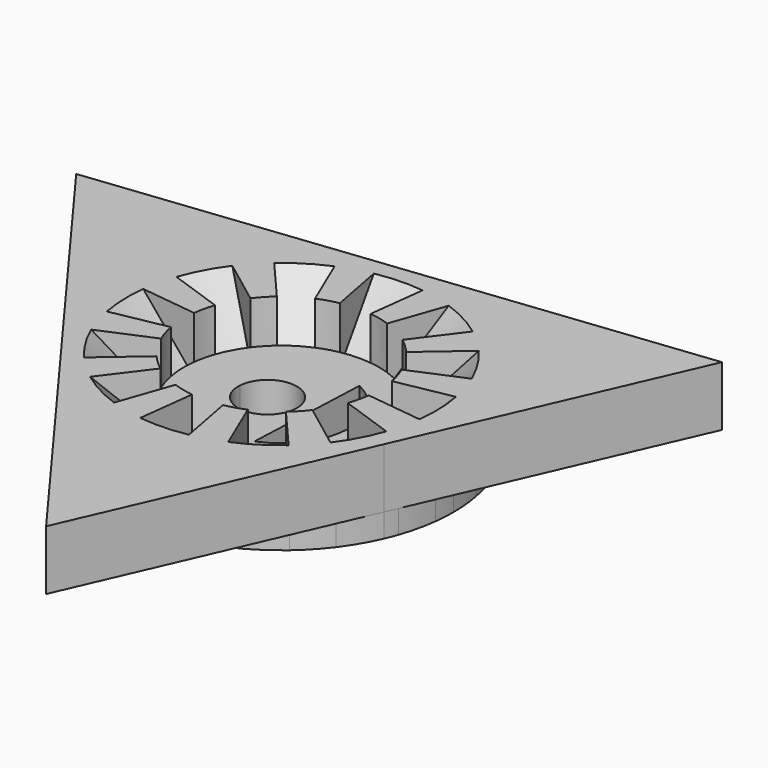
from build123d import *

# Parameters (mm, degrees)
F0_R     = 8.3058
F1_DEPTH = 5.08
F2_SIZE  = 4.826
F4_DEPTH = 5.08
F5_DEPTH = 1.4
F6_DEPTH = 2
F8_DEPTH = 25.4


# Not quite as in the source:
# - a feature names something its author has since deleted; it is built from what else it names


with BuildPart() as f1:
    # F0 (on Top) → F1 (new body)
    with BuildSketch(Plane.XY):
        with BuildLine():
            ThreePointArc((-11.7963555107, -8.6970380191), (-13.4300332581, 5.8674253575), (-1.6336763226, 14.564462754))
            Line((-1.6336763226, 14.564462754), (-26.8600673835, 11.7348487299))
            Line((-26.8600673835, 11.7348487299), (-11.7963555107, -8.6970380191))
        make_face()
        with BuildLine():
            Line((3.2673565821, -29.1289250664), (13.4300329735, -5.8674260091))
            ThreePointArc((13.4300329735, -5.8674260091), (1.6336773074, -14.5644626435), (-11.7963555107, -8.6970380191))
            Line((-11.7963555107, -8.6970380191), (3.2673565821, -29.1289250664))
        make_face()
        with BuildLine():
            ThreePointArc((13.4300329735, -5.8674260091), (14.3460857186, -2.9970482468), (14.6558, 0))
            ThreePointArc((14.6558, 0), (9.768562847, 10.9255504916), (-1.6336763226, 14.564462754))
            ThreePointArc((-1.6336763226, 14.564462754), (-13.4300332581, 5.8674253575), (-11.7963555107, -8.6970380191))
            ThreePointArc((-11.7963555107, -8.6970380191), (1.6336773074, -14.5644626435), (13.4300329735, -5.8674260091))
        make_face()
        Circle(F0_R, mode=Mode.SUBTRACT)
        with BuildLine():
            ThreePointArc((-1.6336763226, 14.564462754), (9.768562847, 10.9255504916), (14.6558, 0))
            ThreePointArc((14.6558, 0), (14.3460857186, -2.9970482468), (13.4300329735, -5.8674260091))
            Line((13.4300329735, -5.8674260091), (23.5927108014, 17.3940763365))
            Line((23.5927108014, 17.3940763365), (-1.6336763226, 14.564462754))
        make_face()
    extrude(amount=F1_DEPTH)

    # F2
    f2_edges = [f1.edges().sort_by_distance(p)[0] for p in [
        (-8.3058, 0, 5.08),
    ]]
    chamfer(f2_edges, length=F2_SIZE)

    # F3 (on face) → F4 (join, through all)
    with BuildSketch(Plane(origin=(0, 0, 0), x_dir=(1, 0, 0), z_dir=(0, 0, -1))):
        with BuildLine():
            ThreePointArc((-8.8120829317, 11.710664714), (-10.0148960998, 10.7002023229), (-11.1026461201, 9.5668031636))
            Line((-11.1026461201, 9.5668031636), (-6.2921408688, 5.4217411343))
            ThreePointArc((-6.2921408688, 5.4217411343), (-5.6756863512, 6.0640661345), (-4.994022736, 6.6367198639))
            Line((-4.994022736, 6.6367198639), (-8.8120829317, 11.710664714))
        make_face()
        with BuildLine():
            ThreePointArc((-2.7382832694, 7.8414359894), (-1.8832554968, 8.0894784983), (-1.0065906245, 8.244579368))
            Line((-1.0065906245, 8.244579368), (-1.7761553221, 14.5477746034))
            ThreePointArc((-1.7761553221, 14.5477746034), (-3.3230532772, 14.2740950871), (-4.8317720074, 13.8364176328))
            Line((-4.8317720074, 13.8364176328), (-2.7382832694, 7.8414359894))
        make_face()
        with BuildLine():
            ThreePointArc((1.5492951207, 8.1600244037), (2.4137921471, 7.9473216313), (3.250556632, 7.6433104884))
            Line((3.250556632, 7.6433104884), (5.7356916717, 13.4868200361))
            ThreePointArc((5.7356916717, 13.4868200361), (4.2591989874, 14.0232556001), (2.7337715126, 14.3985751711))
            Line((2.7337715126, 14.3985751711), (1.5492951207, 8.1600244037))
        make_face()
        with BuildLine():
            ThreePointArc((5.4217411343, 6.2921408688), (6.0640661345, 5.6756863512), (6.6367198639, 4.994022736))
            Line((6.6367198639, 4.994022736), (11.710664714, 8.8120829317))
            ThreePointArc((11.710664714, 8.8120829317), (10.7002023229, 10.0148960998), (9.5668031636, 11.1026461201))
            Line((9.5668031636, 11.1026461201), (5.4217411343, 6.2921408688))
        make_face()
        with BuildLine():
            ThreePointArc((7.8414359894, 2.7382832694), (8.0894784983, 1.8832554968), (8.244579368, 1.0065906245))
            Line((8.244579368, 1.0065906245), (14.5477746034, 1.7761553221))
            ThreePointArc((14.5477746034, 1.7761553221), (14.2740950871, 3.3230532772), (13.8364176328, 4.8317720074))
            Line((13.8364176328, 4.8317720074), (7.8414359894, 2.7382832694))
        make_face()
        with BuildLine():
            Line((14.3985751711, -2.7337715126), (8.1600244037, -1.5492951207))
            ThreePointArc((8.1600244037, -1.5492951207), (7.9473216313, -2.4137921471), (7.6433104884, -3.250556632))
            Line((7.6433104884, -3.250556632), (13.4868200361, -5.7356916717))
            ThreePointArc((13.4868200361, -5.7356916717), (14.0232556001, -4.2591989874), (14.3985751711, -2.7337715126))
        make_face()
        with BuildLine():
            Line((11.1026461201, -9.5668031636), (6.2921408688, -5.4217411343))
            ThreePointArc((6.2921408688, -5.4217411343), (5.6756863512, -6.0640661345), (4.994022736, -6.6367198639))
            Line((4.994022736, -6.6367198639), (8.8120829317, -11.710664714))
            ThreePointArc((8.8120829317, -11.710664714), (10.0148960998, -10.7002023229), (11.1026461201, -9.5668031636))
        make_face()
        with BuildLine():
            Line((4.8317720074, -13.8364176328), (2.7382832694, -7.8414359894))
            ThreePointArc((2.7382832694, -7.8414359894), (1.8832554968, -8.0894784983), (1.0065906245, -8.244579368))
            Line((1.0065906245, -8.244579368), (1.7761553221, -14.5477746034))
            ThreePointArc((1.7761553221, -14.5477746034), (3.3230532772, -14.2740950871), (4.8317720074, -13.8364176328))
        make_face()
        with BuildLine():
            ThreePointArc((-1.5492951207, -8.1600244037), (-2.4137921471, -7.9473216313), (-3.250556632, -7.6433104884))
            Line((-3.250556632, -7.6433104884), (-5.7356916717, -13.4868200361))
            ThreePointArc((-5.7356916717, -13.4868200361), (-4.2591989874, -14.0232556001), (-2.7337715126, -14.3985751711))
            Line((-2.7337715126, -14.3985751711), (-1.5492951207, -8.1600244037))
        make_face()
        with BuildLine():
            Line((-9.5668031636, -11.1026461201), (-5.4217411343, -6.2921408688))
            ThreePointArc((-5.4217411343, -6.2921408688), (-6.0640661345, -5.6756863512), (-6.6367198639, -4.994022736))
            Line((-6.6367198639, -4.994022736), (-11.710664714, -8.8120829317))
            ThreePointArc((-11.710664714, -8.8120829317), (-10.7002023229, -10.0148960998), (-9.5668031636, -11.1026461201))
        make_face()
        with BuildLine():
            Line((-13.8364176328, -4.8317720074), (-7.8414359894, -2.7382832694))
            ThreePointArc((-7.8414359894, -2.7382832694), (-8.0894784983, -1.8832554968), (-8.244579368, -1.0065906245))
            Line((-8.244579368, -1.0065906245), (-14.5477746034, -1.7761553221))
            ThreePointArc((-14.5477746034, -1.7761553221), (-14.2740950871, -3.3230532772), (-13.8364176328, -4.8317720074))
        make_face()
        with BuildLine():
            Line((-7.6433104884, 3.250556632), (-13.4868200361, 5.7356916717))
            ThreePointArc((-13.4868200361, 5.7356916717), (-14.0232556001, 4.2591989874), (-14.3985751711, 2.7337715126))
            Line((-14.3985751711, 2.7337715126), (-8.1600244037, 1.5492951207))
            ThreePointArc((-8.1600244037, 1.5492951207), (-7.9473216313, 2.4137921471), (-7.6433104884, 3.250556632))
        make_face()
    extrude(amount=-F4_DEPTH)


with BuildPart() as f5:
    # F3 (on face) → F5 (new body)
    with BuildSketch(Plane(origin=(0, 0, 0), x_dir=(1, 0, 0), z_dir=(0, 0, -1))):
        with BuildLine():
            ThreePointArc((8.1600244037, -1.5492951207), (8.2692757945, -0.7780690675), (8.3058, 0))
            ThreePointArc((8.3058, 0), (8.2904807145, 0.5042253095), (8.244579368, 1.0065906245))
            ThreePointArc((8.244579368, 1.0065906245), (8.0894784983, 1.8832554968), (7.8414359894, 2.7382832694))
            ThreePointArc((7.8414359894, 2.7382832694), (7.3264138133, 3.9127962221), (6.6367198639, 4.994022736))
            ThreePointArc((6.6367198639, 4.994022736), (6.0640661345, 5.6756863512), (5.4217411343, 6.2921408688))
            ThreePointArc((5.4217411343, 6.2921408688), (4.3884623699, 7.0517878349), (3.250556632, 7.6433104884))
            Line((3.250556632, 7.6433104884), (-3.250556632, -7.6433104884))
            ThreePointArc((-3.250556632, -7.6433104884), (-2.4137921471, -7.9473216313), (-1.5492951207, -8.1600244037))
            ThreePointArc((-1.5492951207, -8.1600244037), (-0.2746259785, -8.301258592), (1.0065906245, -8.244579368))
            ThreePointArc((1.0065906245, -8.244579368), (1.8832554968, -8.0894784983), (2.7382832694, -7.8414359894))
            ThreePointArc((2.7382832694, -7.8414359894), (3.9127962221, -7.3264138133), (4.994022736, -6.6367198639))
            ThreePointArc((4.994022736, -6.6367198639), (5.6756863512, -6.0640661345), (6.2921408688, -5.4217411343))
            ThreePointArc((6.2921408688, -5.4217411343), (7.0517878349, -4.3884623699), (7.6433104884, -3.250556632))
            ThreePointArc((7.6433104884, -3.250556632), (7.9473216313, -2.4137921471), (8.1600244037, -1.5492951207))
        make_face()
        with BuildLine():
            Line((-3.250556632, -7.6433104884), (3.250556632, 7.6433104884))
            ThreePointArc((3.250556632, 7.6433104884), (2.4137921471, 7.9473216313), (1.5492951207, 8.1600244037))
            ThreePointArc((1.5492951207, 8.1600244037), (0.2746259785, 8.301258592), (-1.0065906245, 8.244579368))
            ThreePointArc((-1.0065906245, 8.244579368), (-1.8832554968, 8.0894784983), (-2.7382832694, 7.8414359894))
            ThreePointArc((-2.7382832694, 7.8414359894), (-3.9127962221, 7.3264138133), (-4.994022736, 6.6367198639))
            ThreePointArc((-4.994022736, 6.6367198639), (-5.6756863512, 6.0640661345), (-6.2921408688, 5.4217411343))
            ThreePointArc((-6.2921408688, 5.4217411343), (-7.0517878349, 4.3884623699), (-7.6433104884, 3.250556632))
            ThreePointArc((-7.6433104884, 3.250556632), (-7.9473216313, 2.4137921471), (-8.1600244037, 1.5492951207))
            ThreePointArc((-8.1600244037, 1.5492951207), (-8.301258592, 0.2746259785), (-8.244579368, -1.0065906245))
            ThreePointArc((-8.244579368, -1.0065906245), (-8.0894784983, -1.8832554968), (-7.8414359894, -2.7382832694))
            ThreePointArc((-7.8414359894, -2.7382832694), (-7.3264138133, -3.9127962221), (-6.6367198639, -4.994022736))
            ThreePointArc((-6.6367198639, -4.994022736), (-6.0640661345, -5.6756863512), (-5.4217411343, -6.2921408688))
            ThreePointArc((-5.4217411343, -6.2921408688), (-4.3884623699, -7.0517878349), (-3.250556632, -7.6433104884))
        make_face()
    extrude(amount=-F5_DEPTH)

    # F3 (on face) → F6 (join)
    with BuildSketch(Plane(origin=(0, 0, 0), x_dir=(1, 0, 0), z_dir=(0, 0, -1))):
        with BuildLine():
            ThreePointArc((8.1600244037, -1.5492951207), (8.2692757945, -0.7780690675), (8.3058, 0))
            ThreePointArc((8.3058, 0), (8.2904807145, 0.5042253095), (8.244579368, 1.0065906245))
            ThreePointArc((8.244579368, 1.0065906245), (8.0894784983, 1.8832554968), (7.8414359894, 2.7382832694))
            ThreePointArc((7.8414359894, 2.7382832694), (7.3264138133, 3.9127962221), (6.6367198639, 4.994022736))
            ThreePointArc((6.6367198639, 4.994022736), (6.0640661345, 5.6756863512), (5.4217411343, 6.2921408688))
            ThreePointArc((5.4217411343, 6.2921408688), (4.3884623699, 7.0517878349), (3.250556632, 7.6433104884))
            Line((3.250556632, 7.6433104884), (-3.250556632, -7.6433104884))
            ThreePointArc((-3.250556632, -7.6433104884), (-2.4137921471, -7.9473216313), (-1.5492951207, -8.1600244037))
            ThreePointArc((-1.5492951207, -8.1600244037), (-0.2746259785, -8.301258592), (1.0065906245, -8.244579368))
            ThreePointArc((1.0065906245, -8.244579368), (1.8832554968, -8.0894784983), (2.7382832694, -7.8414359894))
            ThreePointArc((2.7382832694, -7.8414359894), (3.9127962221, -7.3264138133), (4.994022736, -6.6367198639))
            ThreePointArc((4.994022736, -6.6367198639), (5.6756863512, -6.0640661345), (6.2921408688, -5.4217411343))
            ThreePointArc((6.2921408688, -5.4217411343), (7.0517878349, -4.3884623699), (7.6433104884, -3.250556632))
            ThreePointArc((7.6433104884, -3.250556632), (7.9473216313, -2.4137921471), (8.1600244037, -1.5492951207))
        make_face()
        with BuildLine():
            ThreePointArc((8.244579368, 1.0065906245), (8.2904807145, 0.5042253095), (8.3058, 0))
            ThreePointArc((8.3058, 0), (8.2692757945, -0.7780690675), (8.1600244037, -1.5492951207))
            Line((8.1600244037, -1.5492951207), (14.3985751711, -2.7337715126))
            ThreePointArc((14.3985751711, -2.7337715126), (14.5913520901, -1.3729230947), (14.6558, 0))
            ThreePointArc((14.6558, 0), (14.6287687225, 0.8897186654), (14.5477746034, 1.7761553221))
            Line((14.5477746034, 1.7761553221), (8.244579368, 1.0065906245))
        make_face()
        with BuildLine():
            ThreePointArc((7.8414359894, 2.7382832694), (8.0894784983, 1.8832554968), (8.244579368, 1.0065906245))
            Line((8.244579368, 1.0065906245), (14.5477746034, 1.7761553221))
            ThreePointArc((14.5477746034, 1.7761553221), (14.2740950871, 3.3230532772), (13.8364176328, 4.8317720074))
            Line((13.8364176328, 4.8317720074), (7.8414359894, 2.7382832694))
        make_face()
        with BuildLine():
            Line((14.3985751711, -2.7337715126), (8.1600244037, -1.5492951207))
            ThreePointArc((8.1600244037, -1.5492951207), (7.9473216313, -2.4137921471), (7.6433104884, -3.250556632))
            Line((7.6433104884, -3.250556632), (13.4868200361, -5.7356916717))
            ThreePointArc((13.4868200361, -5.7356916717), (14.0232556001, -4.2591989874), (14.3985751711, -2.7337715126))
        make_face()
        with BuildLine():
            ThreePointArc((6.6367198639, 4.994022736), (7.3264138133, 3.9127962221), (7.8414359894, 2.7382832694))
            Line((7.8414359894, 2.7382832694), (13.8364176328, 4.8317720074))
            ThreePointArc((13.8364176328, 4.8317720074), (13.6430563329, 5.3534556632), (13.4300337073, 5.8674243295))
            ThreePointArc((13.4300337073, 5.8674243295), (12.6562803718, 7.3899283347), (11.710664714, 8.8120829317))
            Line((11.710664714, 8.8120829317), (6.6367198639, 4.994022736))
        make_face()
        with BuildLine():
            Line((13.4868200361, -5.7356916717), (7.6433104884, -3.250556632))
            ThreePointArc((7.6433104884, -3.250556632), (7.0517878349, -4.3884623699), (6.2921408688, -5.4217411343))
            Line((6.2921408688, -5.4217411343), (11.1026461201, -9.5668031636))
            ThreePointArc((11.1026461201, -9.5668031636), (12.443062938, -7.7435559249), (13.4868200361, -5.7356916717))
        make_face()
        with BuildLine():
            ThreePointArc((5.4217411343, 6.2921408688), (6.0640661345, 5.6756863512), (6.6367198639, 4.994022736))
            Line((6.6367198639, 4.994022736), (11.710664714, 8.8120829317))
            ThreePointArc((11.710664714, 8.8120829317), (10.7002023229, 10.0148960998), (9.5668031636, 11.1026461201))
            Line((9.5668031636, 11.1026461201), (5.4217411343, 6.2921408688))
        make_face()
        with BuildLine():
            Line((11.1026461201, -9.5668031636), (6.2921408688, -5.4217411343))
            ThreePointArc((6.2921408688, -5.4217411343), (5.6756863512, -6.0640661345), (4.994022736, -6.6367198639))
            Line((4.994022736, -6.6367198639), (8.8120829317, -11.710664714))
            ThreePointArc((8.8120829317, -11.710664714), (10.0148960998, -10.7002023229), (11.1026461201, -9.5668031636))
        make_face()
        with BuildLine():
            ThreePointArc((3.250556632, 7.6433104884), (4.3884623699, 7.0517878349), (5.4217411343, 6.2921408688))
            Line((5.4217411343, 6.2921408688), (9.5668031636, 11.1026461201))
            ThreePointArc((9.5668031636, 11.1026461201), (7.7435559249, 12.443062938), (5.7356916717, 13.4868200361))
            Line((5.7356916717, 13.4868200361), (3.250556632, 7.6433104884))
        make_face()
        with BuildLine():
            Line((8.8120829317, -11.710664714), (4.994022736, -6.6367198639))
            ThreePointArc((4.994022736, -6.6367198639), (3.9127962221, -7.3264138133), (2.7382832694, -7.8414359894))
            Line((2.7382832694, -7.8414359894), (4.8317720074, -13.8364176328))
            ThreePointArc((4.8317720074, -13.8364176328), (6.9042306427, -12.9276476156), (8.8120829317, -11.710664714))
        make_face()
        with BuildLine():
            Line((-3.250556632, -7.6433104884), (3.250556632, 7.6433104884))
            ThreePointArc((3.250556632, 7.6433104884), (2.4137921471, 7.9473216313), (1.5492951207, 8.1600244037))
            ThreePointArc((1.5492951207, 8.1600244037), (0.2746259785, 8.301258592), (-1.0065906245, 8.244579368))
            ThreePointArc((-1.0065906245, 8.244579368), (-1.8832554968, 8.0894784983), (-2.7382832694, 7.8414359894))
            ThreePointArc((-2.7382832694, 7.8414359894), (-3.9127962221, 7.3264138133), (-4.994022736, 6.6367198639))
            ThreePointArc((-4.994022736, 6.6367198639), (-5.6756863512, 6.0640661345), (-6.2921408688, 5.4217411343))
            ThreePointArc((-6.2921408688, 5.4217411343), (-7.0517878349, 4.3884623699), (-7.6433104884, 3.250556632))
            ThreePointArc((-7.6433104884, 3.250556632), (-7.9473216313, 2.4137921471), (-8.1600244037, 1.5492951207))
            ThreePointArc((-8.1600244037, 1.5492951207), (-8.301258592, 0.2746259785), (-8.244579368, -1.0065906245))
            ThreePointArc((-8.244579368, -1.0065906245), (-8.0894784983, -1.8832554968), (-7.8414359894, -2.7382832694))
            ThreePointArc((-7.8414359894, -2.7382832694), (-7.3264138133, -3.9127962221), (-6.6367198639, -4.994022736))
            ThreePointArc((-6.6367198639, -4.994022736), (-6.0640661345, -5.6756863512), (-5.4217411343, -6.2921408688))
            ThreePointArc((-5.4217411343, -6.2921408688), (-4.3884623699, -7.0517878349), (-3.250556632, -7.6433104884))
        make_face()
        with BuildLine():
            ThreePointArc((1.5492951207, 8.1600244037), (2.4137921471, 7.9473216313), (3.250556632, 7.6433104884))
            Line((3.250556632, 7.6433104884), (5.7356916717, 13.4868200361))
            ThreePointArc((5.7356916717, 13.4868200361), (4.2591989874, 14.0232556001), (2.7337715126, 14.3985751711))
            Line((2.7337715126, 14.3985751711), (1.5492951207, 8.1600244037))
        make_face()
        with BuildLine():
            Line((4.8317720074, -13.8364176328), (2.7382832694, -7.8414359894))
            ThreePointArc((2.7382832694, -7.8414359894), (1.8832554968, -8.0894784983), (1.0065906245, -8.244579368))
            Line((1.0065906245, -8.244579368), (1.7761553221, -14.5477746034))
            ThreePointArc((1.7761553221, -14.5477746034), (3.3230532772, -14.2740950871), (4.8317720074, -13.8364176328))
        make_face()
        with BuildLine():
            ThreePointArc((-1.0065906245, 8.244579368), (0.2746259785, 8.301258592), (1.5492951207, 8.1600244037))
            Line((1.5492951207, 8.1600244037), (2.7337715126, 14.3985751711))
            ThreePointArc((2.7337715126, 14.3985751711), (0.4845846776, 14.6477865676), (-1.7761553221, 14.5477746034))
            Line((-1.7761553221, 14.5477746034), (-1.0065906245, 8.244579368))
        make_face()
        with BuildLine():
            Line((-5.7356916717, -13.4868200361), (-3.250556632, -7.6433104884))
            ThreePointArc((-3.250556632, -7.6433104884), (-4.3884623699, -7.0517878349), (-5.4217411343, -6.2921408688))
            Line((-5.4217411343, -6.2921408688), (-9.5668031636, -11.1026461201))
            ThreePointArc((-9.5668031636, -11.1026461201), (-7.7435559249, -12.443062938), (-5.7356916717, -13.4868200361))
        make_face()
        with BuildLine():
            ThreePointArc((-1.5492951207, -8.1600244037), (-2.4137921471, -7.9473216313), (-3.250556632, -7.6433104884))
            Line((-3.250556632, -7.6433104884), (-5.7356916717, -13.4868200361))
            ThreePointArc((-5.7356916717, -13.4868200361), (-4.2591989874, -14.0232556001), (-2.7337715126, -14.3985751711))
            Line((-2.7337715126, -14.3985751711), (-1.5492951207, -8.1600244037))
        make_face()
        with BuildLine():
            ThreePointArc((-2.7337715126, -14.3985751711), (-2.1852995342, -14.4919612056), (-1.6336782694, -14.5644625356))
            ThreePointArc((-1.6336782694, -14.5644625356), (0.0717255143, -14.6556244865), (1.7761553221, -14.5477746034))
            Line((1.7761553221, -14.5477746034), (1.0065906245, -8.244579368))
            ThreePointArc((1.0065906245, -8.244579368), (-0.2746259785, -8.301258592), (-1.5492951207, -8.1600244037))
            Line((-1.5492951207, -8.1600244037), (-2.7337715126, -14.3985751711))
        make_face()
        with BuildLine():
            ThreePointArc((-11.1026461201, 9.5668031636), (-11.4577572909, 9.1385048833), (-11.7963563716, 8.6970368514))
            ThreePointArc((-11.7963563716, 8.6970368514), (-12.728006271, 7.2656954248), (-13.4868200361, 5.7356916717))
            Line((-13.4868200361, 5.7356916717), (-7.6433104884, 3.250556632))
            ThreePointArc((-7.6433104884, 3.250556632), (-7.0517878349, 4.3884623699), (-6.2921408688, 5.4217411343))
            Line((-6.2921408688, 5.4217411343), (-11.1026461201, 9.5668031636))
        make_face()
        with BuildLine():
            ThreePointArc((-2.7382832694, 7.8414359894), (-1.8832554968, 8.0894784983), (-1.0065906245, 8.244579368))
            Line((-1.0065906245, 8.244579368), (-1.7761553221, 14.5477746034))
            ThreePointArc((-1.7761553221, 14.5477746034), (-3.3230532772, 14.2740950871), (-4.8317720074, 13.8364176328))
            Line((-4.8317720074, 13.8364176328), (-2.7382832694, 7.8414359894))
        make_face()
        with BuildLine():
            Line((-9.5668031636, -11.1026461201), (-5.4217411343, -6.2921408688))
            ThreePointArc((-5.4217411343, -6.2921408688), (-6.0640661345, -5.6756863512), (-6.6367198639, -4.994022736))
            Line((-6.6367198639, -4.994022736), (-11.710664714, -8.8120829317))
            ThreePointArc((-11.710664714, -8.8120829317), (-10.7002023229, -10.0148960998), (-9.5668031636, -11.1026461201))
        make_face()
        with BuildLine():
            ThreePointArc((-8.8120829317, 11.710664714), (-10.0148960998, 10.7002023229), (-11.1026461201, 9.5668031636))
            Line((-11.1026461201, 9.5668031636), (-6.2921408688, 5.4217411343))
            ThreePointArc((-6.2921408688, 5.4217411343), (-5.6756863512, 6.0640661345), (-4.994022736, 6.6367198639))
            Line((-4.994022736, 6.6367198639), (-8.8120829317, 11.710664714))
        make_face()
        with BuildLine():
            Line((-7.6433104884, 3.250556632), (-13.4868200361, 5.7356916717))
            ThreePointArc((-13.4868200361, 5.7356916717), (-14.0232556001, 4.2591989874), (-14.3985751711, 2.7337715126))
            Line((-14.3985751711, 2.7337715126), (-8.1600244037, 1.5492951207))
            ThreePointArc((-8.1600244037, 1.5492951207), (-7.9473216313, 2.4137921471), (-7.6433104884, 3.250556632))
        make_face()
        with BuildLine():
            ThreePointArc((-4.994022736, 6.6367198639), (-3.9127962221, 7.3264138133), (-2.7382832694, 7.8414359894))
            Line((-2.7382832694, 7.8414359894), (-4.8317720074, 13.8364176328))
            ThreePointArc((-4.8317720074, 13.8364176328), (-6.9042306427, 12.9276476156), (-8.8120829317, 11.710664714))
            Line((-8.8120829317, 11.710664714), (-4.994022736, 6.6367198639))
        make_face()
        with BuildLine():
            Line((-11.710664714, -8.8120829317), (-6.6367198639, -4.994022736))
            ThreePointArc((-6.6367198639, -4.994022736), (-7.3264138133, -3.9127962221), (-7.8414359894, -2.7382832694))
            Line((-7.8414359894, -2.7382832694), (-13.8364176328, -4.8317720074))
            ThreePointArc((-13.8364176328, -4.8317720074), (-12.9276476156, -6.9042306427), (-11.710664714, -8.8120829317))
        make_face()
        with BuildLine():
            Line((-8.1600244037, 1.5492951207), (-14.3985751711, 2.7337715126))
            ThreePointArc((-14.3985751711, 2.7337715126), (-14.6477865676, 0.4845846776), (-14.5477746034, -1.7761553221))
            Line((-14.5477746034, -1.7761553221), (-8.244579368, -1.0065906245))
            ThreePointArc((-8.244579368, -1.0065906245), (-8.301258592, 0.2746259785), (-8.1600244037, 1.5492951207))
        make_face()
        with BuildLine():
            Line((-13.8364176328, -4.8317720074), (-7.8414359894, -2.7382832694))
            ThreePointArc((-7.8414359894, -2.7382832694), (-8.0894784983, -1.8832554968), (-8.244579368, -1.0065906245))
            Line((-8.244579368, -1.0065906245), (-14.5477746034, -1.7761553221))
            ThreePointArc((-14.5477746034, -1.7761553221), (-14.2740950871, -3.3230532772), (-13.8364176328, -4.8317720074))
        make_face()
    extrude(amount=F6_DEPTH)

    # F7 (on face) → F8 (cut)
    with BuildSketch(Plane.XY.offset(1.4)):
        with BuildLine():
            ThreePointArc((2.0402276918, -5.3927655804), (4.6297015472, -3.4366136274), (5.7524770863, -0.3917358958))
            Line((5.7524770863, -0.3917358958), (2.2578176744, -0.1462228934))
            Line((2.2578176744, -0.1462228934), (2.0402276918, -5.3927655804))
        make_face()
        with BuildLine():
            ThreePointArc((5.7524770863, -0.3917358958), (5.762468309, -0.1959811931), (5.7658, 0))
            ThreePointArc((5.7658, 0), (4.8755646041, 3.0778757985), (2.4797618332, 5.2053079535))
            Line((2.4797618332, 5.2053079535), (2.2578176744, -0.1462228934))
            Line((2.2578176744, -0.1462228934), (5.7524770863, -0.3917358958))
        make_face()
        with BuildLine():
            Line((1.2326478363, -0.0742008462), (-3.7550586709, 0.2762043451))
            ThreePointArc((-3.7550586709, 0.2762043451), (-1.436408013, -2.3928515041), (1.2326478363, -0.0742008462))
        make_face()
        with BuildLine():
            ThreePointArc((1.2387945827, 0.1010017495), (-1.1735502235, 2.5994645903), (-3.7550586709, 0.2762043451))
            Line((-3.7550586709, 0.2762043451), (1.2326478363, -0.0742008462))
            ThreePointArc((1.2326478363, -0.0742008462), (1.2372574235, 0.0133465556), (1.2387945827, 0.1010017495))
        make_face()
    extrude(amount=-F8_DEPTH, mode=Mode.SUBTRACT)


with BuildPart() as f9_1:
    # F9: copy of F1
    add(f1.part)


solid = Compound([f1.part, f5.part])
